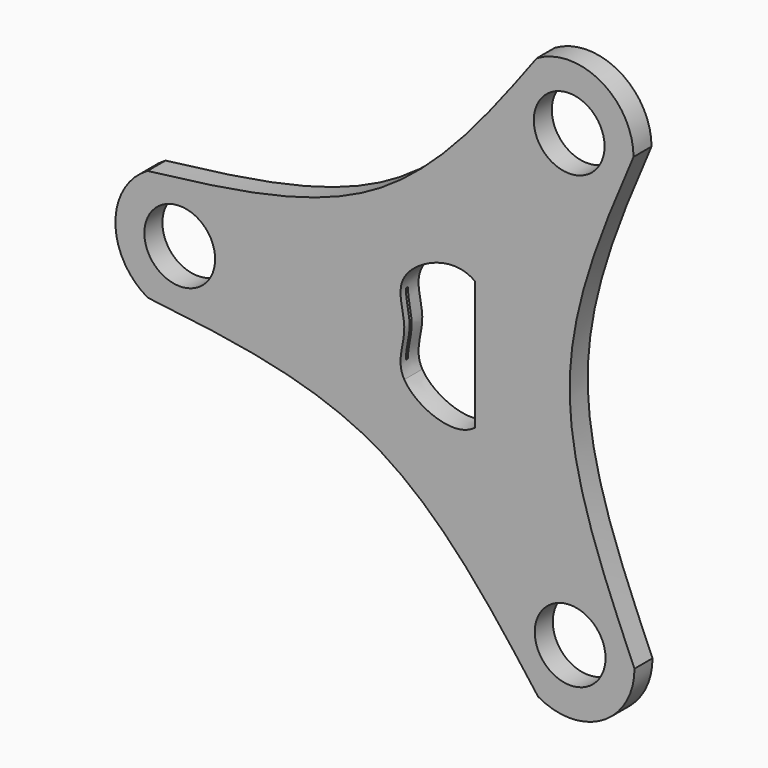
from build123d import *

# Parameters (mm, degrees)
F0_R     = 11
F1_DEPTH = 7
F4_DEPTH = 0.4


with BuildPart() as f1:
    # F0 (on Front) → F1 (new body)
    with BuildSketch(Plane.XZ):
        with BuildLine():
            add(Edge.make_bspline(
                [(-90.8271871838, 17.1252166849), (-65.6361619016, 20.1801984156), (-15.2541113371, 26.2901618769), (15.053487254, 66.9980498131), (30.2072865496, 87.3519937812)],
                knots=[0, 0, 0, 0, 0.5, 1, 1, 1, 1], degree=3))
            ThreePointArc((-90.8271871838, 17.1252166849), (-100.7899149472, -0.2167571218), (-90.7526889605, -17.5157193593))
            add(Edge.make_bspline(
                [(-90.7526889605, -17.5157193593), (-65.5487567691, -20.462322529), (-15.1408923865, -26.3555288685), (15.3415164695, -66.9326828214), (30.5827208975, -87.2212597979)],
                knots=[0, 0, 0, 0, 0.5, 1, 1, 1, 1], degree=3))
            ThreePointArc((30.5827208975, -87.2212597979), (50.5826746476, -87.1782482286), (60.5454024109, -69.8362744219))
            add(Edge.make_bspline(
                [(60.2444662863, 70.096043113), (50.2908494103, 46.7157233653), (30.3950343103, -0.0180945494), (50.4991257729, -46.5724539929), (60.5454024109, -69.8362744219)],
                knots=[0, 0, 0, 0, 0.5002869612, 1, 1, 1, 1], degree=3))
            ThreePointArc((60.2444662863, 70.096043113), (50.2072402996, 87.3950053505), (30.2072865496, 87.3519937812))
        make_face()
        with Locations((-80.7899611971, -0.1737455525)):
            Circle(F0_R, mode=Mode.SUBTRACT)
        with Locations((40.5454486609, -69.8792859912)):
            Circle(F0_R, mode=Mode.SUBTRACT)
        with BuildLine():
            add(Edge.make_bspline(
                [(-11, -14), (-13.6210738364, -9.4558803164), (-8.3789261636, 0), (-16.9662275077, 15.4899287121), (4.2288329874, 25.2994830421), (11, 20)],
                knots=[0, 0, 0, 0, 0.1601841539, 0.3203683079, 0.5248038347, 0.5248038347, 0.5248038347, 0.5248038347], degree=3))
            add(Edge.make_bspline(
                [(11, 20), (19.9679398291, 12.9812032463), (19.9679398291, -12.9812032463), (11, -20)],
                knots=[0.5248038347, 0.5248038347, 0.5248038347, 0.5248038347, 0.7955644732, 0.7955644732, 0.7955644732, 0.7955644732], degree=3))
            add(Edge.make_bspline(
                [(11, -20), (4.2288329874, -25.2994830421), (-7.6548463287, -19.7994469409), (-11, -14)],
                knots=[0.7955644732, 0.7955644732, 0.7955644732, 0.7955644732, 1, 1, 1, 1], degree=3))
        make_face(mode=Mode.SUBTRACT)
        with Locations((40.2445125363, 70.0530315437)):
            Circle(F0_R, mode=Mode.SUBTRACT)
        with BuildLine():
            Line((11, 20), (11, 0))
            Line((11, 0), (11, -20))
            add(Edge.make_bspline(
                [(11, 20), (19.9679398291, 12.9812032463), (19.9679398291, -12.9812032463), (11, -20)],
                knots=[0.5248038347, 0.5248038347, 0.5248038347, 0.5248038347, 0.7955644732, 0.7955644732, 0.7955644732, 0.7955644732], degree=3))
        make_face()
    extrude(amount=F1_DEPTH)

    # F3 (on offset) → F4 (cut, symmetric)
    with BuildSketch(Plane.XZ.offset(4.5)):
        Polygon((-28.5066514462, 9.5), (-28.5066514462, 0), (-28.5066514462, -9.5), (-9.7575942054, -9.85), (-9.7575942054, 0), (-9.7575942054, 9.85), align=None)
    extrude(amount=F4_DEPTH, both=True, mode=Mode.SUBTRACT)


solid = f1.part
